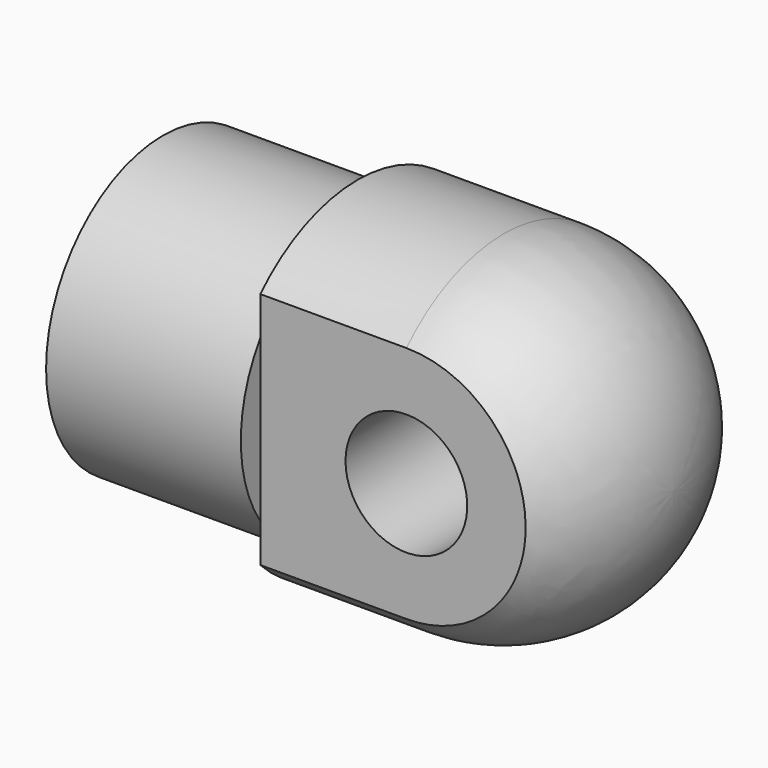
from build123d import *

# Parameters (mm, degrees)
F2_W     = 20
F2_H     = 8.8103966404
F3_DEPTH = 12.5
F4_R     = 2.5
F5_DEPTH = 25


# Not quite as in the source:
# - ends of sketch curves that miss each other by under 0.0002 mm in the source are joined


with BuildPart() as f1:
    # F0 (on Top) → F1 (revolve)
    with BuildSketch(Plane.XY):
        with BuildLine():
            Line((0, 6), (0, 2))
            Line((0, 2), (8, 2))
            Line((8, 2), (8, 0))
            Line((8, 0), (21, 0))
            ThreePointArc((21, 0), (18.9497474683, 4.9497475801), (14, 7.0000001118))
            Line((14, 7.0000001118), (8, 7.0000001118))
            Line((8, 7.0000001118), (8, 6))
            Line((8, 6), (0, 6))
        make_face()
    revolve(axis=Axis((-4.767620936, 0, 0), (-1, 0, 0)))

    # F2 (on Top) → F3 (cut, symmetric)
    with BuildSketch(Plane.XY):
        with Locations((18, -9.4051983202)):
            Rectangle(F2_W, F2_H)
        with Locations((18, 9.4051983202)):
            Rectangle(F2_W, F2_H)
    extrude(amount=F3_DEPTH, both=True, mode=Mode.SUBTRACT)

    # F4 (on face) → F5 (cut)
    with BuildSketch(Plane(origin=(0, 5, 0), x_dir=(-1, 0, 0), z_dir=(0, 1, 0))):
        with Locations((-14, 0)):
            Circle(F4_R)
    extrude(amount=-F5_DEPTH, mode=Mode.SUBTRACT)


solid = f1.part
